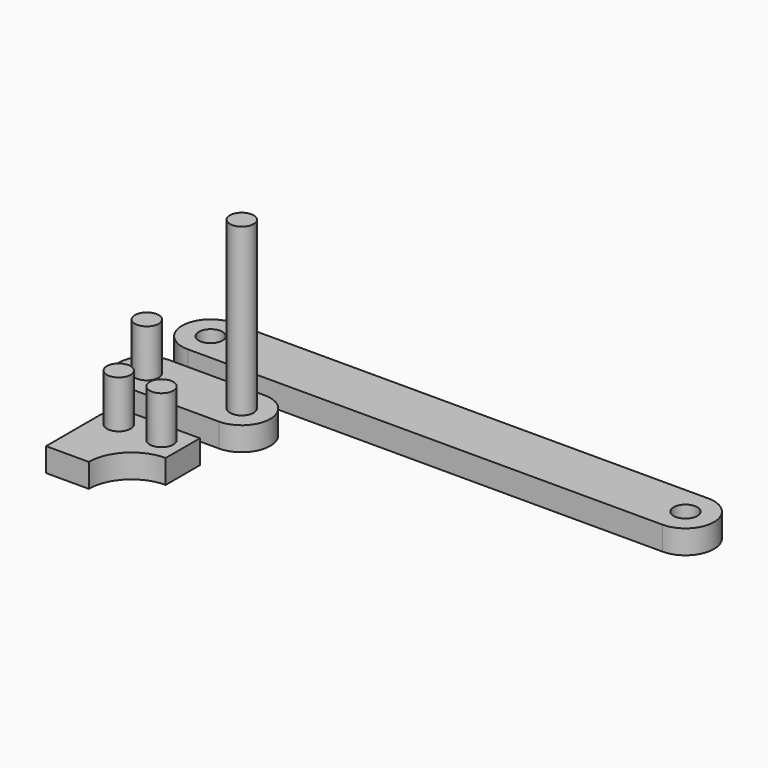
from build123d import *

# Parameters (mm, degrees)
F0_R     = 12.5
F1_DEPTH = 25
F2_DEPTH = 200
F3_DEPTH = 75
F4_DEPTH = 25
F5_R     = 44.99999
F6_R     = 20
F7_DEPTH = 75
F8_DEPTH = 25


# Not quite as in the source:
# - a fillet or chamfer is up to 0.001 mm smaller than in the source, because OpenCascade refuses the exact size


with BuildPart() as f1:
    # F0 (on Top) → F1 (new body)
    with BuildSketch(Plane.XY):
        with BuildLine():
            ThreePointArc((50, -30), (80, 0), (50, 30))
            Line((50, 30), (-50, 30))
            ThreePointArc((-50, 30), (-80, 0), (-50, -30))
            Line((-50, -30), (50, -30))
        make_face()
        with Locations((-50, 0)):
            Circle(F0_R, mode=Mode.SUBTRACT)
        with Locations((50, 0)):
            Circle(F0_R, mode=Mode.SUBTRACT)
    extrude(amount=F1_DEPTH)

    # F0 (on Top) → F2 (join)
    with BuildSketch(Plane.XY):
        with Locations((50, 0)):
            Circle(F0_R)
    extrude(amount=F2_DEPTH)

    # F0 (on Top) → F3 (join)
    with BuildSketch(Plane.XY):
        with Locations((-50, 0)):
            Circle(F0_R)
    extrude(amount=F3_DEPTH)


with BuildPart() as f4:
    # F0 (on Top) → F4 (new body)
    with BuildSketch(Plane.XY):
        Polygon((56.2614613771, -107.9339570552), (56.2614613771, -62.9339570552), (-33.7385386229, -62.9339570552), (-33.7385386229, -152.9339570552), (11.2614613771, -152.9339570552), (11.2614613771, -107.9339570552), align=None)
        with Locations((-11.2385386229, -85.4339570552)):
            Circle(F0_R, mode=Mode.SUBTRACT)
        with Locations((33.7614613771, -85.4339570552)):
            Circle(F0_R, mode=Mode.SUBTRACT)
    extrude(amount=F4_DEPTH)

    # F5 (radius 45 in the source; OpenCascade refuses exactly that, so slightly less here)
    f5_edges = [f4.edges().sort_by_distance(p)[0] for p in [
        (11.261461, -107.933957, 12.5),
    ]]
    fillet(f5_edges, radius=F5_R)

    # F6
    f6_edges = [f4.edges().sort_by_distance(p)[0] for p in [
        (-33.738539, -62.933957, 12.5),
    ]]
    fillet(f6_edges, radius=F6_R)

    # F0 (on Top) → F7 (join)
    with BuildSketch(Plane.XY):
        with Locations((-11.2385386229, -85.4339570552)):
            Circle(F0_R)
        with Locations((33.7614613771, -85.4339570552)):
            Circle(F0_R)
    extrude(amount=F7_DEPTH)


with BuildPart() as f8:
    # F0 (on Top) → F8 (new body)
    with BuildSketch(Plane.XY):
        with BuildLine():
            ThreePointArc((449.5936667547, 54.4830423594), (479.5936667547, 84.4830423594), (449.5936667547, 114.4830423594))
            Line((449.5936667547, 114.4830423594), (-50.4063332453, 114.4830423594))
            ThreePointArc((-50.4063332453, 114.4830423594), (-80.4063332453, 84.4830423594), (-50.4063332453, 54.4830423594))
            Line((-50.4063332453, 54.4830423594), (449.5936667547, 54.4830423594))
        make_face()
        with Locations((-50.4063332453, 84.4830423594)):
            Circle(F0_R, mode=Mode.SUBTRACT)
        with Locations((449.5936667547, 84.4830423594)):
            Circle(F0_R, mode=Mode.SUBTRACT)
    extrude(amount=F8_DEPTH)


solid = Compound([f1.part, f4.part, f8.part])
